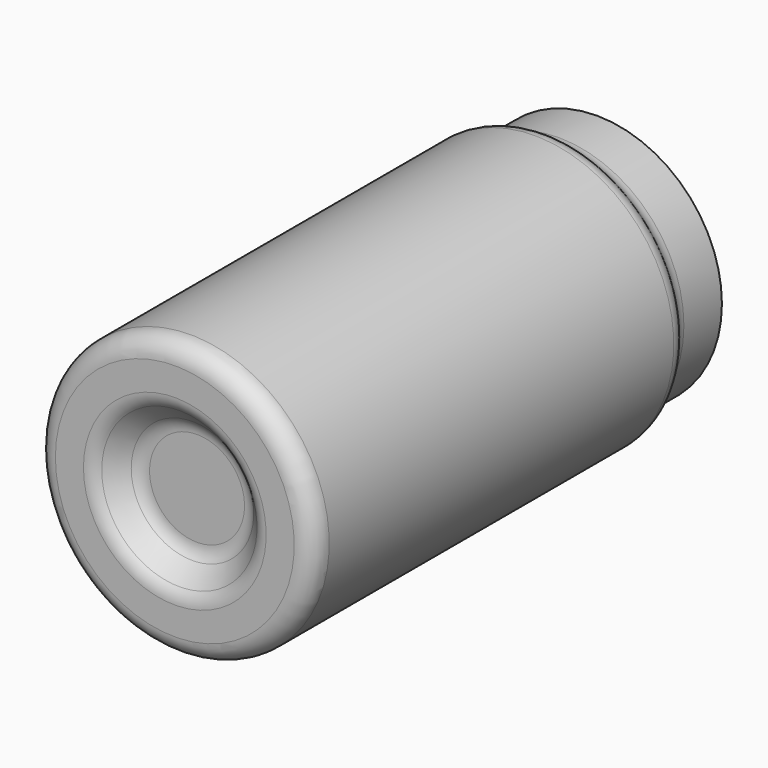
from build123d import *


# Not quite as in the source:
# - ends of sketch curves that miss each other by under 0.0002 mm in the source are joined


with BuildPart() as f1:
    # F0 (on Top) → F1 (revolve)
    with BuildSketch(Plane.XY):
        with BuildLine():
            Line((-50, 0), (-49.25, 0))
            Line((-49.25, 0), (-49.25, 67.100505))
            ThreePointArc((-49.25, 67.100505), (-48.7742470782, 69.4922764523), (-47.4194173824, 71.5199223824))
            Line((-47.4194173824, 71.5199223824), (-46.519922, 72.419417))
            ThreePointArc((-46.519922, 72.419417), (-44.839933623, 74.9336983992), (-44.25, 77.899495))
            Line((-44.25, 77.899495), (-44.25, 95))
            Line((-44.25, 95), (-45, 95))
            Line((-45, 95), (-45, 77.899495))
            ThreePointArc((-45, 77.899495), (-45.5328434077, 75.2207106468), (-47.0502530317, 72.9497470317))
            Line((-47.0502530317, 72.9497470317), (-47.949748, 72.050252))
            ThreePointArc((-47.949748, 72.050252), (-49.4671568629, 69.7792886999), (-50, 67.100505))
            Line((-50, 67.100505), (-50, 0))
        make_face()
        with BuildLine():
            Line((0, -85), (0, -84.25))
            Line((0, -84.25), (-17.100505, -84.25))
            ThreePointArc((-17.100505, -84.25), (-20.0663019275, -84.8399337583), (-22.5805830542, -86.5199229458))
            Line((-22.5805830542, -86.5199229458), (-28.480078, -92.419418))
            ThreePointArc((-28.480078, -92.419418), (-30.5077238744, -93.7742472135), (-32.899495, -94.25))
            Line((-32.899495, -94.25), (-43, -94.25))
            ThreePointArc((-43, -94.25), (-47.4194173824, -92.4194173824), (-49.25, -88))
            Line((-49.25, -88), (-49.25, 0))
            Line((-49.25, 0), (-50, 0))
            Line((-50, 0), (-50, -88))
            ThreePointArc((-50, -88), (-47.9497474683, -92.9497474683), (-43, -95))
            Line((-43, -95), (-32.899495, -95))
            ThreePointArc((-32.899495, -95), (-30.2207113001, -94.4671568629), (-27.9497480317, -92.9497479683))
            Line((-27.9497480317, -92.9497479683), (-22.050253, -87.050253))
            ThreePointArc((-22.050253, -87.050253), (-19.7792893532, -85.5328434077), (-17.100505, -85))
            Line((-17.100505, -85), (0, -85))
        make_face()
    revolve(axis=Axis((0, 0, 0), (0, -1, 0)))


solid = f1.part
